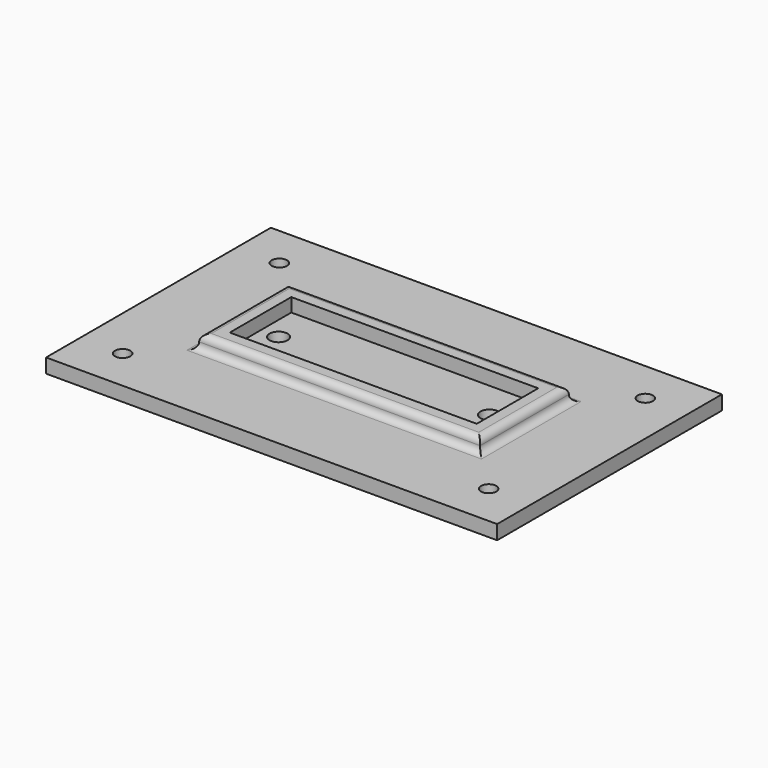
from build123d import *

# Parameters (mm, degrees)
F1_W     = 132.6
F1_H     = 82.6
F1_R     = 2.25
F2_DEPTH = 4.2
F0_W     = 82.6
F0_H     = 32.6
F0_W_2   = 72.6
F0_H_2   = 22.6
F3_DEPTH = 4
F4_R     = 2.655
F5_DEPTH = 3.8
F5_TAPER = 1.6
F6_R     = 1.75
F7_DEPTH = 4.201
F8_R     = 1.99999


# Not quite as in the source:
# - a fillet or chamfer is up to 0.001 mm smaller than in the source, because OpenCascade refuses the exact size


with BuildPart() as f2:
    # F1 (on Top) → F2 (new body)
    with BuildSketch(Plane.XY):
        Rectangle(F1_W, F1_H)
        with Locations((-53.8, -28.8)):
            Circle(F1_R, mode=Mode.SUBTRACT)
        with Locations((53.8, -28.8)):
            Circle(F1_R, mode=Mode.SUBTRACT)
        with Locations((-53.8, 28.8)):
            Circle(F1_R, mode=Mode.SUBTRACT)
        with Locations((53.8, 28.8)):
            Circle(F1_R, mode=Mode.SUBTRACT)
    extrude(amount=-F2_DEPTH)

    # F0 (on Top) → F3 (join)
    with BuildSketch(Plane.XY):
        Rectangle(F0_W, F0_H)
        Rectangle(F0_W_2, F0_H_2, mode=Mode.SUBTRACT)
    extrude(amount=F3_DEPTH)

    # F4 (on face) → F5 (cut)
    with BuildSketch(Plane.XY):
        with Locations((-31, 0)):
            Circle(F4_R)
        with Locations((31, 0)):
            Circle(F4_R)
    extrude(amount=-F5_DEPTH, taper=F5_TAPER, mode=Mode.SUBTRACT)

    # F6 (on face) → F7 (cut, through all)
    with BuildSketch(Plane.XY):
        with Locations((31, 0)):
            Circle(F6_R)
        with Locations((-31, 0)):
            Circle(F6_R)
    extrude(amount=-F7_DEPTH, mode=Mode.SUBTRACT)

    # F8 (radius 2 in the source; OpenCascade refuses exactly that, so slightly less here)
    f8_edges = [f2.edges().sort_by_distance(p)[0] for p in [
        (0, 16.3, 0),
        (-41.3, 0, 0),
        (0, -16.3, 0),
        (41.3, 0, 0),
        (0, -16.3, 4),
        (41.3, 0, 4),
        (0, 16.3, 4),
        (-41.3, 0, 4),
    ]]
    fillet(f8_edges, radius=F8_R)


solid = f2.part
